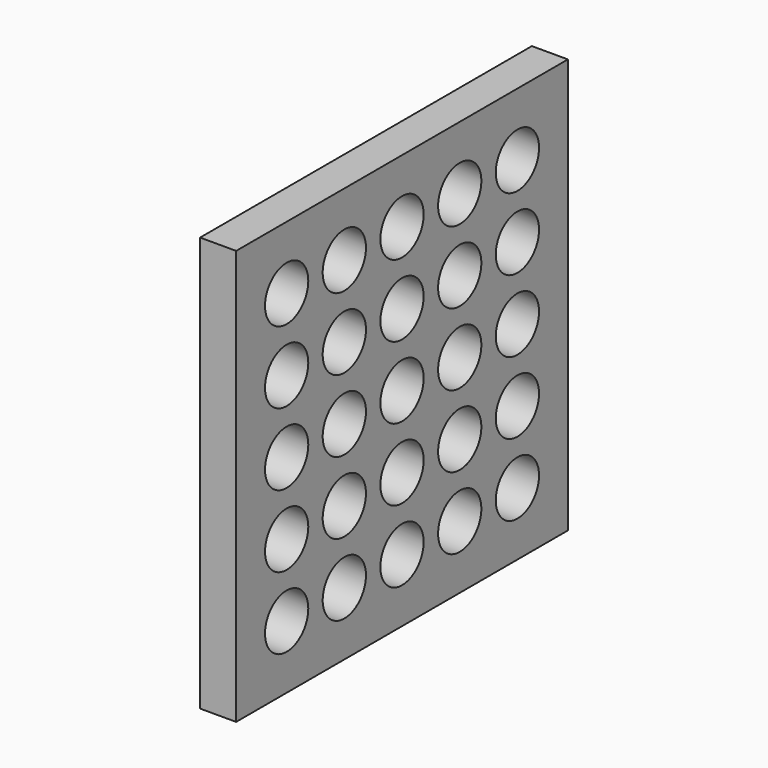
from build123d import *

# Parameters (mm, degrees)
F0_R     = 0.75
F1_DEPTH = 1


# Not quite as in the source:
# - a feature names something its author has since deleted; it is built from what else it names


with BuildPart() as f1:
    # F0 (on Right) → F1 (new body)
    with BuildSketch(Plane.YZ):
        Polygon((8.384144865, 0), (0, 0), (0, -11.5), (11.5, -11.5), (11.5, 0), (10.38414, 0), (9.5, 0), align=None)
        with Locations((1.75, -9.75)):
            Circle(F0_R, mode=Mode.SUBTRACT)
        with Locations((1.75, -7.75)):
            Circle(F0_R, mode=Mode.SUBTRACT)
        with Locations((3.75, -9.75)):
            Circle(F0_R, mode=Mode.SUBTRACT)
        with Locations((3.75, -7.75)):
            Circle(F0_R, mode=Mode.SUBTRACT)
        with Locations((1.75, -5.75)):
            Circle(F0_R, mode=Mode.SUBTRACT)
        with Locations((1.75, -3.75)):
            Circle(F0_R, mode=Mode.SUBTRACT)
        with Locations((1.75, -1.75)):
            Circle(F0_R, mode=Mode.SUBTRACT)
        with Locations((3.75, -5.75)):
            Circle(F0_R, mode=Mode.SUBTRACT)
        with Locations((3.75, -3.75)):
            Circle(F0_R, mode=Mode.SUBTRACT)
        with Locations((3.75, -1.75)):
            Circle(F0_R, mode=Mode.SUBTRACT)
        with Locations((5.75, -9.75)):
            Circle(F0_R, mode=Mode.SUBTRACT)
        with Locations((7.75, -9.75)):
            Circle(F0_R, mode=Mode.SUBTRACT)
        with Locations((5.75, -7.75)):
            Circle(F0_R, mode=Mode.SUBTRACT)
        with Locations((7.75, -7.75)):
            Circle(F0_R, mode=Mode.SUBTRACT)
        with Locations((9.75, -9.75)):
            Circle(F0_R, mode=Mode.SUBTRACT)
        with Locations((9.75, -7.75)):
            Circle(F0_R, mode=Mode.SUBTRACT)
        with Locations((5.75, -5.75)):
            Circle(F0_R, mode=Mode.SUBTRACT)
        with Locations((5.75, -3.75)):
            Circle(F0_R, mode=Mode.SUBTRACT)
        with Locations((7.75, -5.75)):
            Circle(F0_R, mode=Mode.SUBTRACT)
        with Locations((7.75, -3.75)):
            Circle(F0_R, mode=Mode.SUBTRACT)
        with Locations((5.75, -1.75)):
            Circle(F0_R, mode=Mode.SUBTRACT)
        with Locations((7.75, -1.75)):
            Circle(F0_R, mode=Mode.SUBTRACT)
        with Locations((9.75, -5.75)):
            Circle(F0_R, mode=Mode.SUBTRACT)
        with Locations((9.75, -3.75)):
            Circle(F0_R, mode=Mode.SUBTRACT)
        with Locations((9.75, -1.75)):
            Circle(F0_R, mode=Mode.SUBTRACT)
    extrude(amount=F1_DEPTH)


solid = f1.part
